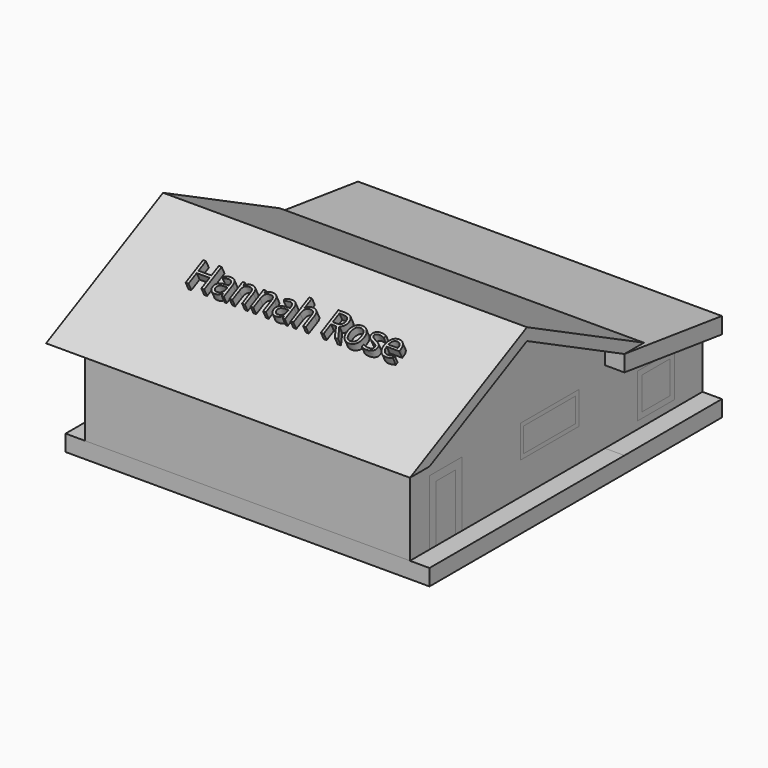
from build123d import *

# Parameters (mm, degrees)
F0_W         = 228.6
F0_H         = 101.6
F0_W_2       = 144.7796318314
F0_H_2       = 137.1599945068
F1_DEPTH     = 508
F0_W_3       = 76.2
F0_H_3       = 177.8
F2_DEPTH     = 508
F0_W_4       = 203.2000002861
F0_H_4       = 76.2000002861
F0_W_5       = 109.2196373245
F3_DEPTH     = 508
F4_DEPTH     = 568.96
F5_TEXT_SIZE = 107.0511216919
F6_DEPTH     = 25.4


# Not quite as in the source:
# - Text() gives the source's letters only with a copy of the font that has no kerning and outlines rounded to 1/6400 em; it was checked with that copy


with BuildPart() as f1:
    # F0 (on Right) → F1 (new body, symmetric)
    with BuildSketch(Plane.YZ):
        Polygon((-381, 0), (0, 0), (0, 190.5), align=None)
        Polygon((0, 190.5), (0, 0), (381, 0), align=None)
        Polygon((381, 0), (0, 0), (-381, 0), (-381, -279.4), (-304.8, -279.4), (-304.8, -76.2), (-177.8, -76.2), (-177.8, -279.4), (381, -279.4), (381, -50.8), align=None)
        with Locations((165.1, -127)):
            Rectangle(F0_W, F0_H, mode=Mode.SUBTRACT)
        Polygon((761.999634578, -101.072315), (381, -50.8), (381, -279.4), (761.999634578, -278.872315), align=None)
        with Locations((580.3898159157, -187.377767471)):
            Rectangle(F0_W_2, F0_H_2, mode=Mode.SUBTRACT)
    extrude(amount=F1_DEPTH, both=True)


with BuildPart() as f2:
    # F0 (on Right) → F2 (new body, symmetric)
    with BuildSketch(Plane.YZ):
        with Locations((-241.3, -190.5)):
            Rectangle(F0_W_3, F0_H_3)
    extrude(amount=F2_DEPTH, both=True)


with BuildPart() as f2b:
    # F0 (on Right) → F2, piece 2 (new body, symmetric)
    with BuildSketch(Plane.YZ):
        with Locations((165.1, -127)):
            Rectangle(F0_W_4, F0_H_4)
    extrude(amount=F2_DEPTH, both=True)


with BuildPart() as f2c:
    # F0 (on Right) → F2, piece 3 (new body, symmetric)
    with BuildSketch(Plane.YZ):
        with Locations((580.3898159157, -187.377767471)):
            Rectangle(F0_W_5, F0_H)
    extrude(amount=F2_DEPTH, both=True)


with BuildPart() as f3:
    # F0 (on Right) → F3 (new body, symmetric)
    with BuildSketch(Plane.YZ):
        Polygon((-304.8, -76.2), (-304.8, -279.4), (-279.4, -279.4), (-279.4, -101.6), (-203.2, -101.6), (-203.2, -279.4), (-177.8, -279.4), (-177.8, -76.2), align=None)
    extrude(amount=F3_DEPTH, both=True)


with BuildPart() as f3b:
    # F0 (on Right) → F3, piece 2 (new body, symmetric)
    with BuildSketch(Plane.YZ):
        with Locations((580.3898159157, -187.377767471)):
            Rectangle(F0_W_2, F0_H_2)
        with Locations((580.3898159157, -187.377767471)):
            Rectangle(F0_W_5, F0_H, mode=Mode.SUBTRACT)
    extrude(amount=F3_DEPTH, both=True)


with BuildPart() as f3c:
    # F0 (on Right) → F3, piece 3 (new body, symmetric)
    with BuildSketch(Plane.YZ):
        with Locations((165.1, -127)):
            Rectangle(F0_W, F0_H)
        with Locations((165.1, -127)):
            Rectangle(F0_W_4, F0_H_4, mode=Mode.SUBTRACT)
    extrude(amount=F3_DEPTH, both=True)


with BuildPart() as f4:
    # F0 (on Right) → F4 (new body, symmetric)
    with BuildSketch(Plane.YZ):
        Polygon((-457.2, 0), (-381, 0), (0, 190.5), (0, 228.6), align=None)
        Polygon((0, 190.5), (381, 0), (457.2, 0), (0, 228.6), align=None)
    extrude(amount=F4_DEPTH, both=True)

    # F5 (on face) → F6 (join)
    with BuildSketch(Plane(origin=(0, -91.44, 182.88), x_dir=(1, 0, 0), z_dir=(0, -0.4472135955, 0.894427191))):
        with Locations((-335.5505615473, -127.2900570184)):
            Text('Hannah Rose', F5_TEXT_SIZE, font='Open Sans', text_align=(TextAlign.LEFT, TextAlign.BOTTOM))
    extrude(amount=F6_DEPTH)


with BuildPart() as f4b:
    # F0 (on Right) → F4, piece 2 (new body, symmetric)
    with BuildSketch(Plane.YZ):
        Polygon((761.999634578, -50.272315), (381, 0), (381, -50.8), (761.999634578, -101.072315), align=None)
    extrude(amount=F4_DEPTH, both=True)


with BuildPart() as f4c:
    # F0 (on Right) → F4, piece 3 (new body, symmetric)
    with BuildSketch(Plane.YZ):
        Polygon((761.999634578, -278.872315), (381, -279.4), (381, -330.2), (762.069992578, -329.6722662771), align=None)
        Polygon((-304.8, -279.4), (-381, -279.4), (-381, -330.2), (381, -330.2), (381, -279.4), (-177.8, -279.4), (-203.2, -279.4), (-279.4, -279.4), align=None)
    extrude(amount=F4_DEPTH, both=True)


solid = Compound([f1.part, f2.part, f2b.part, f2c.part, f3.part, f3b.part, f3c.part, f4.part, f4b.part, f4c.part])
